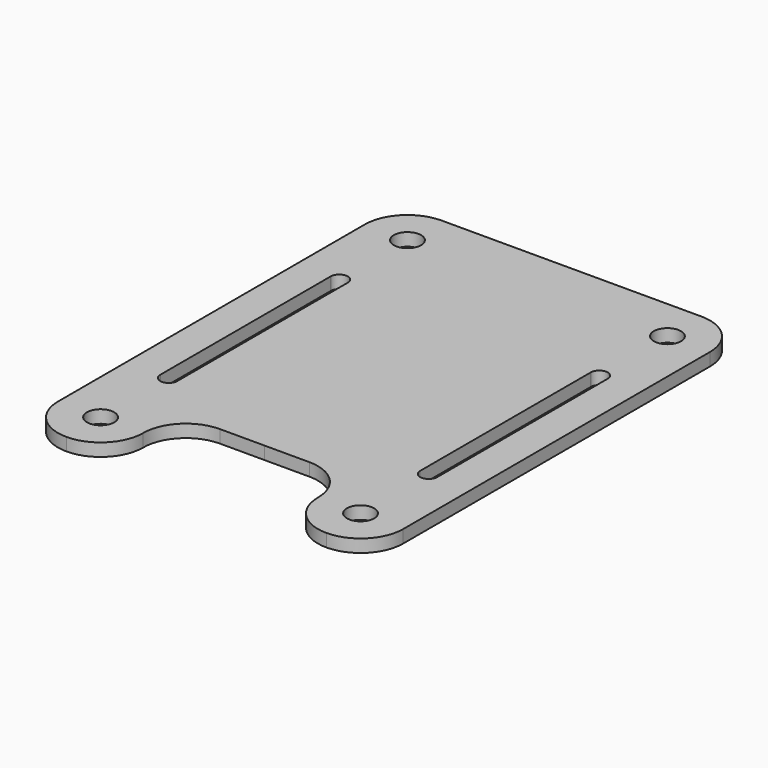
from build123d import *
from build123d import SkipClean  # not in build123d's __all__

# Parameters (mm, degrees)
F0_R     = 1.6
F1_DEPTH = 1.5
F3_DEPTH = 25
F5_DEPTH = 25


# Not quite as in the source:
# - a pattern or mirror of a feature is missing from the dataset's text; its kind, count and spacing are read off the source's solid


with BuildPart() as f1:
    # F0 (on Top) → F1 (new body)
    with BuildSketch(Plane.XY):
        with BuildLine():
            ThreePointArc((20.25, 22.5), (18.7855339059, 26.0355339059), (15.25, 27.5))
            Line((15.25, 27.5), (-15.25, 27.5))
            ThreePointArc((-15.25, 27.5), (-18.7855339059, 26.0355339059), (-20.25, 22.5))
            Line((-20.25, 22.5), (-20.25, -22.5))
            ThreePointArc((-20.25, -22.5), (-18.7855339059, -26.0355339059), (-15.25, -27.5))
            Line((-15.25, -27.5), (15.25, -27.5))
            ThreePointArc((15.25, -27.5), (18.7855339059, -26.0355339059), (20.25, -22.5))
            Line((20.25, -22.5), (20.25, 22.5))
        make_face()
        with Locations((-15.25, -22.5)):
            Circle(F0_R, mode=Mode.SUBTRACT)
        with Locations((15.25, -22.5)):
            Circle(F0_R, mode=Mode.SUBTRACT)
        with Locations((-15.25, 22.5)):
            Circle(F0_R, mode=Mode.SUBTRACT)
        with Locations((15.25, 22.5)):
            Circle(F0_R, mode=Mode.SUBTRACT)
    extrude(amount=F1_DEPTH)

    # F2 (on face) → F3 (cut)
    with BuildSketch(Plane.XY.offset(1.5)):
        with BuildLine():
            Line((-14.2506566552, 12.5362336746), (-14.2506547559, 12.4638187474))
            ThreePointArc((-14.2506547559, 12.4638187474), (-14.2500000003, 12.5000262282), (-14.2506566552, 12.5362336746))
        make_face()
        with BuildLine():
            Line((-14.2500000003, -12.4999737718), (-14.2506547559, 12.4638187474))
            Line((-14.2506547559, 12.4638187474), (-14.2506566552, 12.5362336746))
            ThreePointArc((-14.2506566552, 12.5362336746), (-15.2591368155, 13.4999582584), (-16.2498385848, 12.5179667556))
            Line((-16.2498385848, 12.5179667556), (-16.2498388166, 12.4820461463))
            Line((-16.2498388166, 12.4820461463), (-16.25, -12.499993548))
            ThreePointArc((-16.25, -12.499993548), (-15.2499901119, -13.5), (-14.2500000003, -12.4999737718))
        make_face()
        with BuildLine():
            Line((-16.2498388166, 12.4820461463), (-16.2498385848, 12.5179667556))
            ThreePointArc((-16.2498385848, 12.5179667556), (-16.25, 12.500006452), (-16.2498388166, 12.4820461463))
        make_face()
    f3 = extrude(amount=-F3_DEPTH, mode=Mode.SUBTRACT)

    # F3_copies: F3 across plane
    add(f3.mirror(Plane(origin=(0, 0, 0), x_dir=(0, 0, 1), z_dir=(1, 0, 0))), clean=False, mode=Mode.SUBTRACT)

    # F4 (on face) → F5 (cut)
    with BuildSketch(Plane.XY.offset(1.5)):
        with BuildLine():
            Line((5.2500000017, -17.5), (9e-10, -17.5))
            Line((9e-10, -17.5), (0, -27.5))
            Line((0, -27.5), (0, -33.427875489))
            Line((0, -33.427875489), (15.25, -33.427875489))
            Line((15.25, -33.427875489), (15.25, -27.5))
            ThreePointArc((15.2500000017, -27.5), (11.7144660958, -26.0355339059), (10.2500000017, -22.5))
            ThreePointArc((10.2500000017, -22.5), (8.7855339077, -18.9644660941), (5.2500000017, -17.5))
        make_face()
    f5 = extrude(amount=-F5_DEPTH, mode=Mode.SUBTRACT)

    # F5_copies: F5 across plane
    with SkipClean():  # cleaning this boolean's faces spoils the solid; the shape is the same uncleaned
        add(f5.mirror(Plane(origin=(0, 0, 0), x_dir=(0, 0, -1), z_dir=(-1, 0, 0))), clean=False, mode=Mode.SUBTRACT)


solid = f1.part
